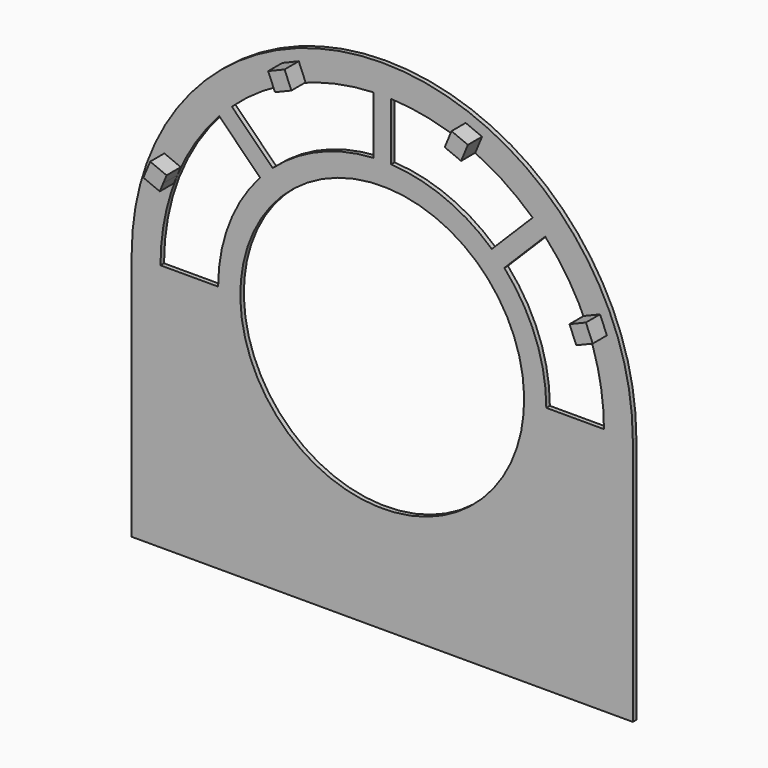
from build123d import *

# Parameters (mm, degrees)
F1_DEPTH = 12.7
F3_DEPTH = 50.8


# Not quite as in the source:
# - a feature names something its author has since deleted; it is built from what else it names


with BuildPart() as f1:
    # F0 (on Front) → F1 (new body)
    with BuildSketch(Plane.XZ):
        with BuildLine():
            ThreePointArc((-95.1022987413, 273.3746719669), (60.4202481719, 242.4393139794), (192.265897133, 154.3428678411))
            Line((192.265897133, 154.3428678411), (412.2821720991, 374.3591428073))
            ThreePointArc((412.2821720992, 374.3591428073), (-95.1022987413, 584.5246719669), (-602.4867695817, 374.3591428072))
            Line((-602.4867695817, 374.3591428073), (-382.4704946155, 154.3428678411))
            ThreePointArc((-382.4704946155, 154.3428678411), (-250.6248456544, 242.4393139794), (-95.1022987413, 273.3746719669))
        make_face()
        with BuildLine():
            ThreePointArc((-525.7952385086, 333.5886362184), (-338.1062782931, 453.6381751115), (-120.5022987413, 501.4664686041))
            Line((-120.5022987413, 501.4664686041), (-120.5022987413, 336.1876832954))
            ThreePointArc((-120.5022987413, 336.1876832954), (-274.9252436096, 301.1056642939), (-408.9254886305, 216.7188863404))
            Line((-408.9254886305, 216.7188863404), (-525.7952385086, 333.5886362184))
        make_face(mode=Mode.SUBTRACT)
        with BuildLine():
            Line((-69.7022987413, 336.1876832954), (-69.7022987413, 501.4664686041))
            ThreePointArc((-69.7022987413, 501.4664686041), (147.9016808106, 453.6381751115), (335.5906410261, 333.5886362184))
            Line((335.5906410261, 333.5886362184), (218.720891148, 216.7188863404))
            ThreePointArc((218.720891148, 216.7188863404), (84.7206461271, 301.1056642939), (-69.7022987413, 336.1876832954))
        make_face(mode=Mode.SUBTRACT)
        with BuildLine():
            ThreePointArc((192.265897133, 154.3428678411), (280.3623432713, 22.49721888), (311.2977012587, -133.0253280331))
            ThreePointArc((311.2977012587, -133.0253280331), (-250.6248456544, -508.4899700457), (-382.4704946155, 154.3428678411))
            Line((-382.4704946155, 154.3428678411), (-602.4867695817, 374.3591428073))
            ThreePointArc((-602.4867695817, 374.3591428072), (-758.0320572947, 141.5691688604), (-812.6522987413, -133.0253280331))
            Line((-812.6522987413, -133.0253280331), (-812.6522987413, -844.2450938398))
            Line((-812.6522987413, -844.2450938398), (0, -844.2450938398))
            Line((0, -844.2450938398), (622.4477012587, -844.2450938398))
            Line((622.4477012587, -844.2450938398), (622.4477012587, -133.0253280331))
            ThreePointArc((622.4477012587, -133.0253280331), (567.8274598122, 141.5691688604), (412.2821720992, 374.3591428073))
            Line((412.2821720991, 374.3591428073), (192.265897133, 154.3428678411))
        make_face()
        with BuildLine():
            ThreePointArc((-444.8465131148, 180.7978618561), (-533.9364452785, 34.9943191303), (-565.0022987413, -133.0253280331))
            Line((-565.0022987413, -133.0253280331), (-730.1022987413, -133.0253280331))
            ThreePointArc((-730.1022987413, -133.0253280331), (-686.5094627576, 98.1944080408), (-561.7162629929, 297.6676117342))
            Line((-561.7162629929, 297.6676117342), (-444.8465131148, 180.7978618561))
        make_face(mode=Mode.SUBTRACT)
        with BuildLine():
            ThreePointArc((371.5116655103, 297.6676117342), (496.3048652751, 98.1944080408), (539.8977012587, -133.0253280331))
            Line((539.8977012587, -133.0253280331), (374.7977012587, -133.0253280331))
            ThreePointArc((374.7977012587, -133.0253280331), (343.731847796, 34.9943191303), (254.6419156323, 180.7978618561))
            Line((254.6419156323, 180.7978618561), (371.5116655103, 297.6676117342))
        make_face(mode=Mode.SUBTRACT)
    extrude(amount=F1_DEPTH)

    # F2 (on face) → F3 (join)
    with BuildSketch(Plane.XZ.offset(12.7)):
        Polygon((-691.485961068, 86.5121113929), (-681.7658018859, 109.9786515187), (-672.0456427039, 133.4451916445), (-718.9787229554, 152.8855100086), (-738.4190413196, 105.952429757), align=None)
        Polygon((528.7741254729, 152.8855100086), (481.8410452213, 133.4451916445), (491.5612025764, 109.9786559296), (501.2813635855, 86.5121113929), (548.2144438371, 105.952429757), align=None)
        Polygon((-381.013136783, 490.851096181), (-361.5728184189, 443.9180159294), (-338.1062857272, 453.6381720322), (-314.6397381673, 463.3583342936), (-334.0800565315, 510.2914145452), align=None)
        Polygon((143.8754590489, 510.2914145452), (124.4351406848, 463.3583342936), (147.9016748411, 453.6381775841), (171.3682209364, 443.9180159294), (190.8085393005, 490.851096181), align=None)
    extrude(amount=F3_DEPTH)


solid = f1.part
